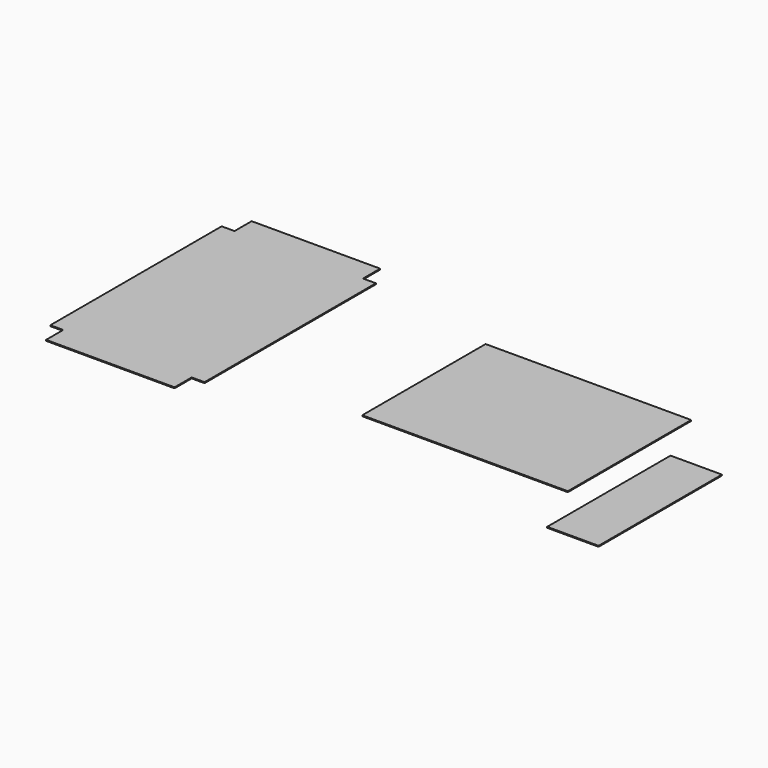
from build123d import *

# Parameters (mm, degrees)
F1_DEPTH = 5.55625
F0_W     = 1219.2
F0_H     = 914.4
F2_DEPTH = 5.55625
F0_W_2   = 304.8
F3_DEPTH = 5.55625


# Not quite as in the source:
# - a length typed as a fraction of an inch, garbled in the dataset ("3 / 203.2 mm" for 3/8 in), is restored


with BuildPart() as f1:
    # F0 (on Top) → F1 (new body)
    with BuildSketch(Plane.XY):
        Polygon((3107.6152240753, 866.6990060806), (3107.6152240753, 739.6990060806), (3869.6152240753, 739.6990060806), (3869.6152240753, 866.6990060806), (3945.8152240753, 866.6990060806), (3945.8152240753, 2136.6990060806), (3869.6152240753, 2136.6990060806), (3869.6152240753, 2263.6990060806), (3107.6152240753, 2263.6990060806), (3107.6152240753, 2136.6990060806), (3031.4152240753, 2136.6990060806), (3031.4152240753, 866.6990060806), align=None)
    extrude(amount=F1_DEPTH)


with BuildPart() as f2:
    # F0 (on Top) → F2 (new body)
    with BuildSketch(Plane.XY):
        with Locations((5332.9943939209, 1521.108457756)):
            Rectangle(F0_W, F0_H)
    extrude(amount=F2_DEPTH)


with BuildPart() as f3:
    # F0 (on Top) → F3 (new body)
    with BuildSketch(Plane.XY):
        with Locations((6243.4768508911, 1182.3549363136)):
            Rectangle(F0_W_2, F0_H)
    extrude(amount=F3_DEPTH)


solid = Compound([f1.part, f2.part, f3.part])
